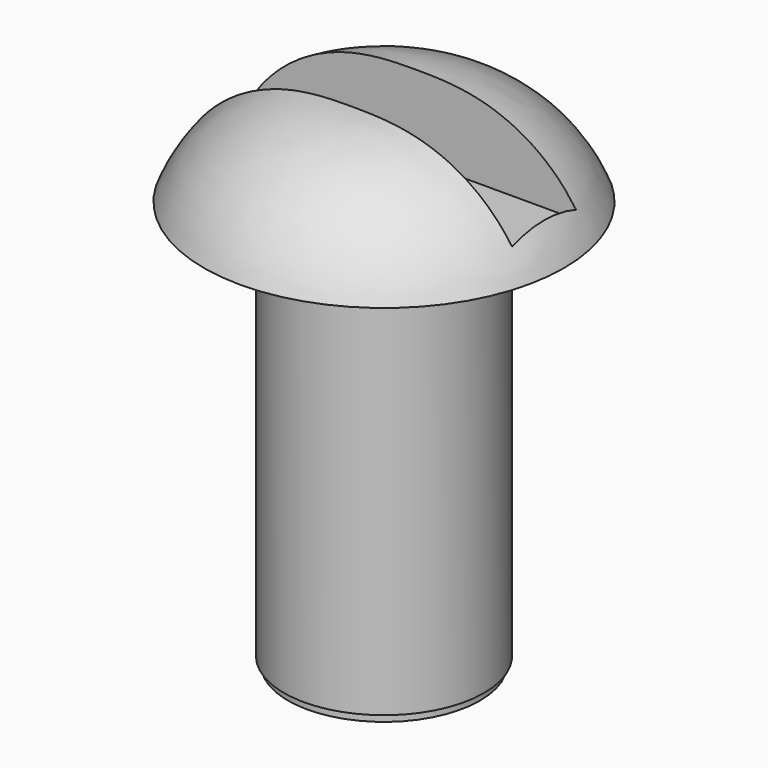
from build123d import *

# Parameters (mm, degrees)
F2_R     = 5.715
F3_DEPTH = 3.175
F5_W     = 10.16
F5_H     = 2.54
F6_DEPTH = 2.54
F0_R     = 3.175
F7_DEPTH = 12.7
F8_R     = 3.048
F9_DEPTH = 0.254


# Not quite as in the source:
# - a fillet or chamfer that OpenCascade refuses, or shapes differently, is made with other operations: its cross-section is extruded or revolved along the edge and cut away or added


with BuildPart() as f3:
    # F2 (on offset) → F3 (new body)
    with BuildSketch(Plane.XY.offset(12.7)):
        Circle(F2_R)
    extrude(amount=F3_DEPTH)

    # F4: fillet of radius 5.08 on 1 edges, made by hand

    # F4_s1 → F4_t2 (revolve, cut)
    with BuildSketch(Plane.XZ):
        with BuildLine():
            ThreePointArc((5.715, 12.7), (3.8455202921, 15.0071134838), (1.0057139607, 15.875))
            Line((1.0057139607, 15.875), (5.715, 15.875))
            Line((5.715, 15.875), (5.715, 12.7))
        make_face()
    revolve(axis=Axis((0, 0, 15.875), (0, 0, 1)), mode=Mode.SUBTRACT)

    # F5 (on face) → F6 (cut)
    with BuildSketch(Plane.XY.offset(15.875)):
        Rectangle(F5_W, F5_H)
    extrude(amount=-F6_DEPTH, mode=Mode.SUBTRACT)


with BuildPart() as f7:
    # F0 (on Top) → F7 (new body)
    with BuildSketch(Plane.XY):
        Circle(F0_R)
    extrude(amount=F7_DEPTH)

    # F8 (on face) → F9 (join)
    with BuildSketch(Plane(origin=(0, 0, 0), x_dir=(1, 0, 0), z_dir=(0, 0, -1))):
        Circle(F8_R)
    extrude(amount=F9_DEPTH)


solid = Compound([f3.part, f7.part])
